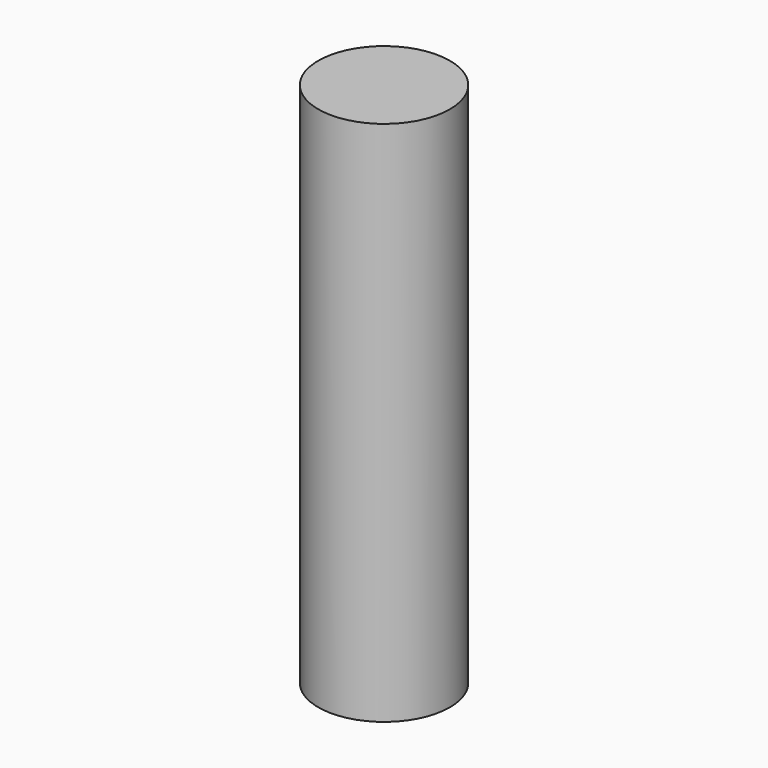
from build123d import *

# Parameters (mm, degrees)
F0_R     = 12.7
F1_DEPTH = 101.6


# Not quite as in the source:
# - a feature of the source that left no trace in its solid (it failed there, or was rolled back) is left out


with BuildPart() as f1:
    # F0 (on Top) → F1 (new body)
    with BuildSketch(Plane.XY):
        Circle(F0_R)
    extrude(amount=F1_DEPTH)


solid = f1.part
